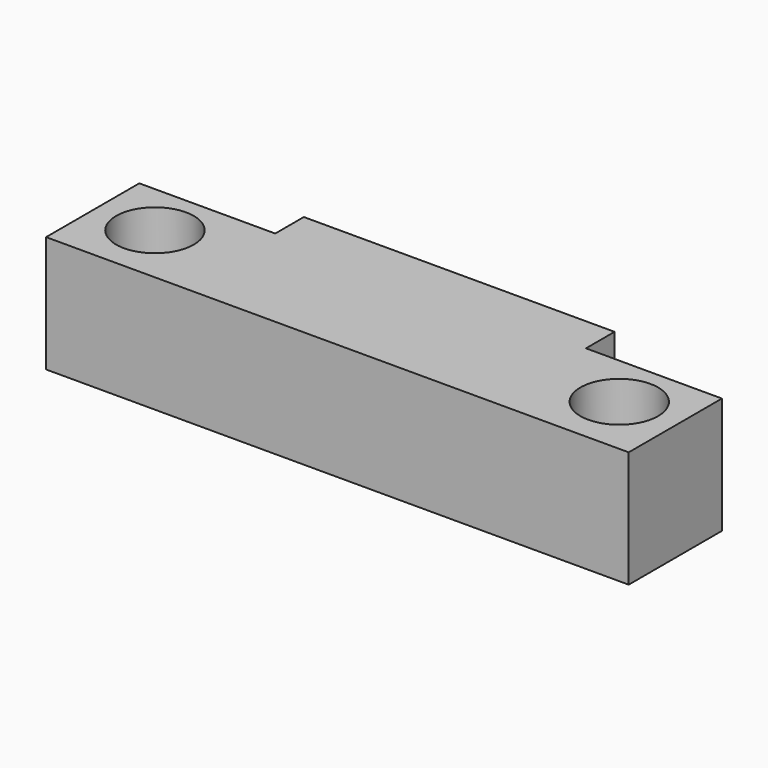
from build123d import *

# Parameters (mm, degrees)
F0_R     = 5
F1_DEPTH = 15
F3_R     = 1.5
F3_R_2   = 1
F4_DEPTH = 26


# Not quite as in the source:
# - a feature names something its author has since deleted; it is built from what else it names


with BuildPart() as f1:
    # F0 (on Top) → F1 (new body)
    with BuildSketch(Plane.XY):
        Polygon((-37.5, 9.6315789474), (-37.5, -5.3684210526), (37.5, -5.3684210526), (37.5, 9.6315789474), (20, 9.6315789474), (20, 14.2315789474), (-20, 14.2315789474), (-20, 9.6315789474), align=None)
        with Locations((-29.8843569823, 2.6315789474)):
            Circle(F0_R, mode=Mode.SUBTRACT)
        with Locations((29.8843569823, 2.6315789474)):
            Circle(F0_R, mode=Mode.SUBTRACT)
    extrude(amount=F1_DEPTH)

    # F3 (on offset) → F4 (join, symmetric)
    with BuildSketch(Plane(origin=(0, 0, 0), x_dir=(0, -1, 0), z_dir=(-1, 0, 0))):
        with Locations((-15.7305789474, 1)):
            Circle(F3_R)
        with Locations((-15.7305789474, 1)):
            Circle(F3_R_2, mode=Mode.SUBTRACT)
    extrude(amount=F4_DEPTH, both=True)


solid = f1.part
